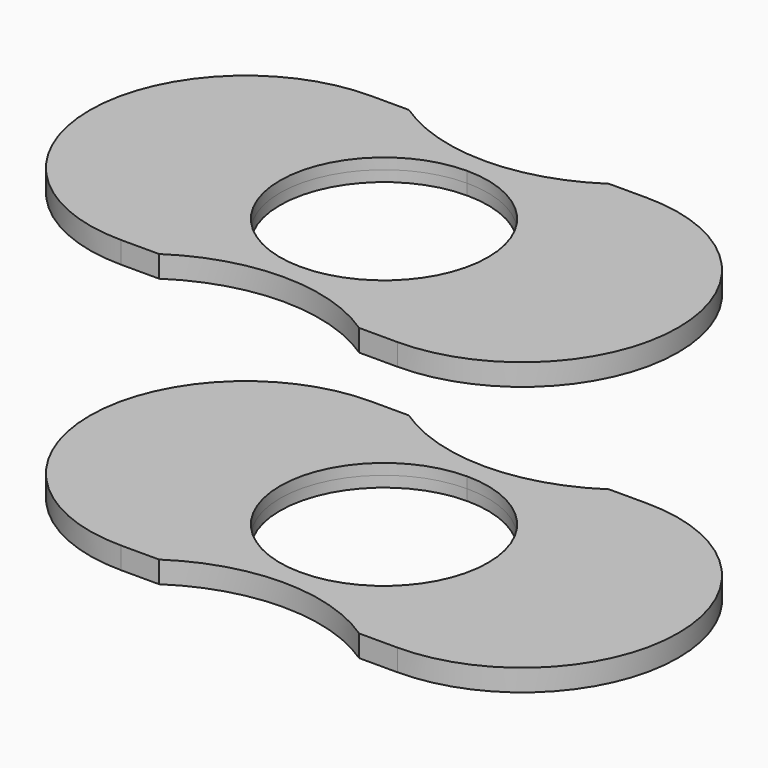
from build123d import *

# Parameters (mm, degrees)
F1_DEPTH = 1.15


# Not quite as in the source:
# - a feature names something its author has since deleted; it is built from what else it names


with BuildPart() as f1:
    # F0 (on Top) → F1 (new body, symmetric)
    with BuildSketch(Plane.XY):
        with BuildLine():
            Line((0, 11), (0, 13.2910696268))
            ThreePointArc((0, 13.2910696268), (-5.5299040268, 14.1136066175), (-10.5810132518, 16.51))
            Line((-10.5810132518, 16.51), (-14.6177952834, 16.51))
            ThreePointArc((-14.6177952834, 16.51), (-22.0869562882, 14.7238491531), (-27.94, 9.7518696408))
            Line((-27.94, 9.7518696408), (-27.94, -9.7518696408))
            ThreePointArc((-27.94, -9.7518696408), (-22.0869562882, -14.7238491531), (-14.6177952834, -16.51))
            Line((-14.6177952834, -16.51), (-10.5810132518, -16.51))
            ThreePointArc((-10.5810132518, -16.51), (-5.5299040268, -14.1136066175), (0, -13.2910696268))
            Line((0, -13.2910696268), (0, -11))
            ThreePointArc((0, -11), (-11, 0), (0, 11))
        make_face()
        with BuildLine():
            ThreePointArc((27.94, 9.7518696408), (22.0869562882, 14.7238491531), (14.6177952834, 16.51))
            Line((14.6177952834, 16.51), (10.5810132518, 16.51))
            ThreePointArc((10.5810132518, 16.51), (5.5299040268, 14.1136066175), (0, 13.2910696268))
            Line((0, 13.2910696268), (0, 11))
            ThreePointArc((0, 11), (7.7781745931, 7.7781745931), (11, 0))
            ThreePointArc((11, 0), (7.7781745931, -7.7781745931), (0, -11))
            Line((0, -11), (0, -13.2910696268))
            ThreePointArc((0, -13.2910696268), (5.5299040268, -14.1136066175), (10.5810132518, -16.51))
            Line((10.5810132518, -16.51), (14.6177952834, -16.51))
            ThreePointArc((14.6177952834, -16.51), (22.0869562882, -14.7238491531), (27.94, -9.7518696408))
            Line((27.94, -9.7518696408), (27.94, 9.7518696408))
        make_face()
        with BuildLine():
            ThreePointArc((27.94, -9.7518696408), (31.1277952834, 0), (27.94, 9.7518696408))
            Line((27.94, 9.7518696408), (27.94, -9.7518696408))
        make_face()
        with BuildLine():
            Line((-27.94, -9.7518696408), (-27.94, 9.7518696408))
            ThreePointArc((-27.94, 9.7518696408), (-31.1277952834, 0), (-27.94, -9.7518696408))
        make_face()
    extrude(amount=F1_DEPTH, both=True)


with BuildPart() as f2_1:
    # F2: copy of F1
    add(f1.part.moved(Location((0, 0, 28.448))))


solid = Compound([f1.part, f2_1.part])
